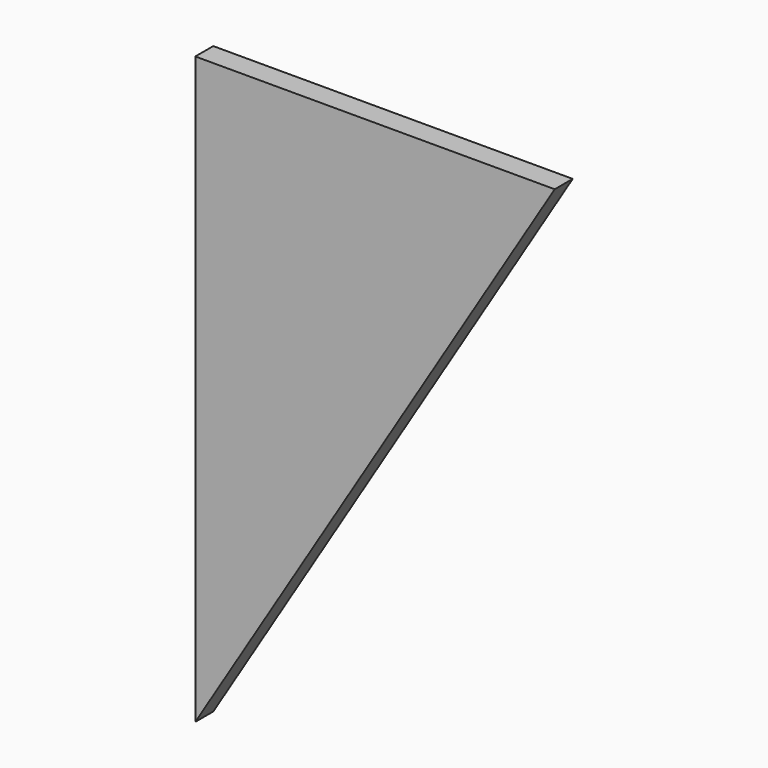
from build123d import *

# Parameters (mm, degrees)
F1_DEPTH = 3.175


# Not quite as in the source:
# - a length typed as a fraction of an inch, garbled in the dataset ("3 / 203.2 mm" for 3/8 in), is restored


with BuildPart() as f1:
    # F0 (on Front) → F1 (new body)
    with BuildSketch(Plane.XZ):
        Polygon((50.8, 0), (0, 0), (0, -82.79384), align=None)
    extrude(amount=F1_DEPTH)


solid = f1.part
